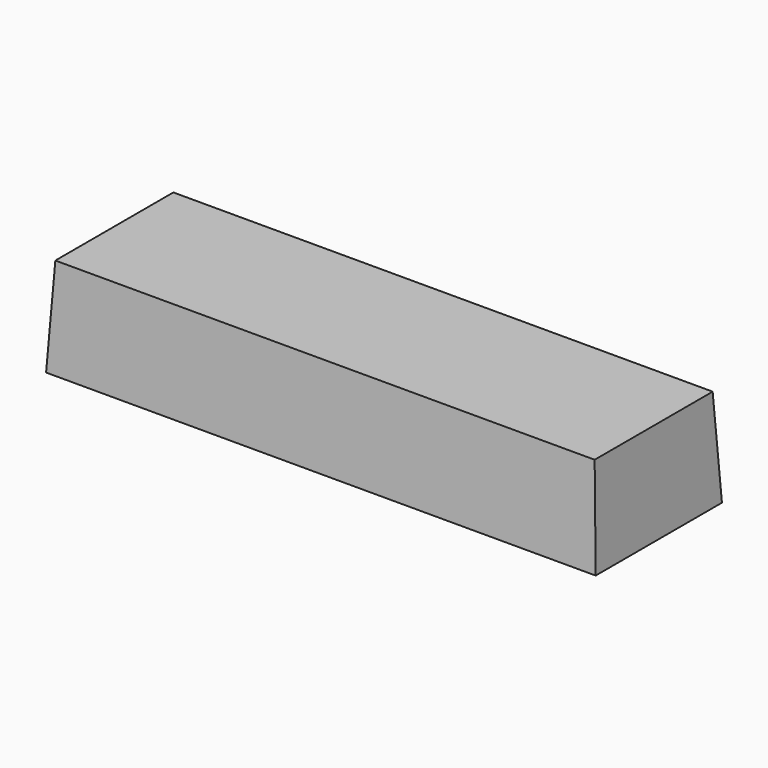
from build123d import *

# Parameters (mm, degrees)
F0_W     = 139.4754946232
F0_H     = 38.145236671
F1_DEPTH = 25.4
F1_TAPER = -3


with BuildPart() as f1:
    # F0 (on Top) → F1 (new body)
    with BuildSketch(Plane.XY):
        with Locations((69.7377473116, 19.0726183355)):
            Rectangle(F0_W, F0_H)
    extrude(amount=-F1_DEPTH, taper=F1_TAPER)


solid = f1.part
